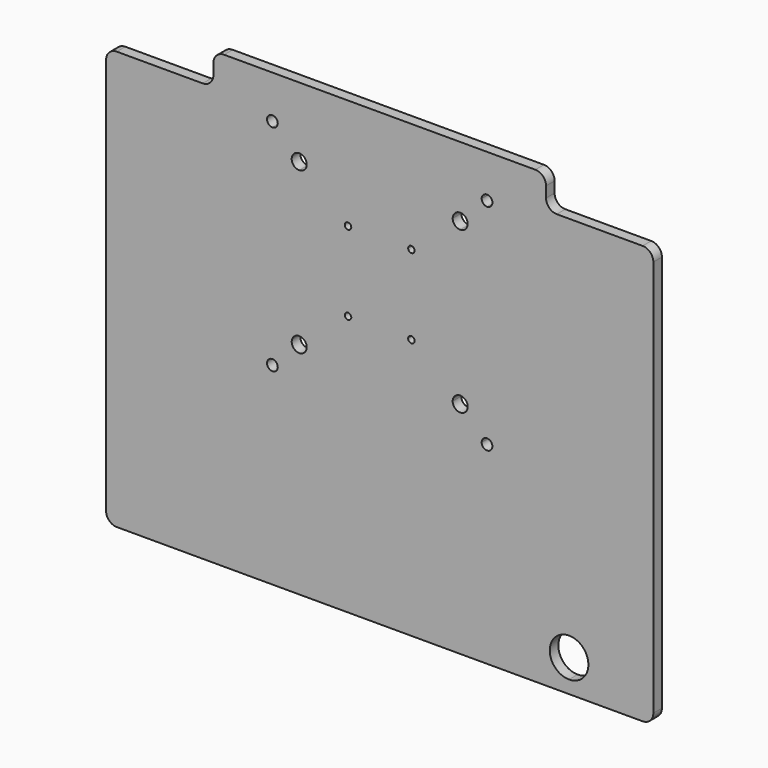
from build123d import *

# Parameters (mm, degrees)
F1_DEPTH = 5


with BuildPart() as f1:
    # F0 (on Front) → F1 (new body)
    with BuildSketch(Plane.XZ):
        with BuildLine():
            Line((88.225863874, -105), (122.5, -105))
            ThreePointArc((122.5, -105), (126.0355339059, -103.5355339059), (127.5, -100))
            Line((127.5, -100), (127.5, 85))
            ThreePointArc((127.5, 85), (126.0355339059, 88.5355339059), (122.5, 90))
            Line((122.5, 90), (82.5, 90))
            ThreePointArc((82.5, 90), (78.9644660941, 91.4644660941), (77.5, 95))
            Line((77.5, 95), (77.5, 100))
            ThreePointArc((77.5, 100), (76.0355339059, 103.5355339059), (72.5, 105))
            Line((72.5, 105), (0, 105))
            Line((0, 105), (-72.5, 105))
            ThreePointArc((-72.5, 105), (-76.0355339059, 103.5355339059), (-77.5, 100))
            Line((-77.5, 100), (-77.5, 95))
            ThreePointArc((-77.5, 95), (-78.9644660941, 91.4644660941), (-82.5, 90))
            Line((-82.5, 90), (-122.5, 90))
            ThreePointArc((-122.5, 90), (-126.0355339059, 88.5355339059), (-127.5, 85))
            Line((-127.5, 85), (-127.5, -100))
            ThreePointArc((-127.5, -100), (-126.0355339059, -103.5355339059), (-122.5, -105))
            Line((-122.5, -105), (88.225863874, -105))
        make_face()
        with BuildLine():
            ThreePointArc((97.225863874, -90), (94.5898249046, -96.3639610307), (88.225863874, -99))
            ThreePointArc((88.225863874, -99), (81.8619028433, -83.6360389693), (97.225863874, -90))
        make_face(mode=Mode.SUBTRACT)
        with BuildLine():
            Line((-47.5, 85), (0, 85))
            Line((0, 85), (47.5, 85))
            ThreePointArc((47.5, 85), (50, 87.5), (52.5, 85))
            ThreePointArc((52.5, 85), (51.767766953, 83.232233047), (50, 82.5))
            Line((50, 82.5), (50, -12.5))
            ThreePointArc((50, -12.5), (51.767766953, -13.232233047), (52.5, -15))
            ThreePointArc((52.5, -15), (50, -17.5), (47.5, -15))
            Line((47.5, -15), (-47.5, -15))
            ThreePointArc((-47.5, -15), (-51.767766953, -16.767766953), (-50, -12.5))
            Line((-50, -12.5), (-50, 82.5))
            ThreePointArc((-50, 82.5), (-51.767766953, 86.767766953), (-47.5, 85))
        make_face(mode=Mode.SUBTRACT)
        with BuildLine():
            Line((47.5, 85), (0, 85))
            Line((0, 85), (-47.5, 85))
            ThreePointArc((-47.5, 85), (-48.232233047, 83.232233047), (-50, 82.5))
            Line((-50, 82.5), (-50, -12.5))
            ThreePointArc((-50, -12.5), (-48.232233047, -13.232233047), (-47.5, -15))
            Line((-47.5, -15), (47.5, -15))
            ThreePointArc((47.5, -15), (48.232233047, -13.232233047), (50, -12.5))
            Line((50, -12.5), (50, 82.5))
            ThreePointArc((50, 82.5), (48.232233047, 83.232233047), (47.5, 85))
        make_face()
        with BuildLine():
            Line((34, -2.5), (-34, -2.5))
            ThreePointArc((-34, -2.5), (-39.9748737342, -4.9748737342), (-37.5, 1))
            Line((-37.5, 1), (-37.5, 69))
            ThreePointArc((-37.5, 69), (-39.9748737342, 74.9748737342), (-34, 72.5))
            Line((-34, 72.5), (34, 72.5))
            ThreePointArc((34, 72.5), (37.5, 76), (41, 72.5))
            ThreePointArc((41, 72.5), (39.9748737342, 70.0251262658), (37.5, 69))
            Line((37.5, 69), (37.5, 1))
            ThreePointArc((37.5, 1), (39.9748737342, -0.0251262658), (41, -2.5))
            ThreePointArc((41, -2.5), (37.5, -6), (34, -2.5))
        make_face(mode=Mode.SUBTRACT)
        with BuildLine():
            ThreePointArc((-37.5, 1), (-35.0251262658, -0.0251262658), (-34, -2.5))
            Line((-34, -2.5), (34, -2.5))
            ThreePointArc((34, -2.5), (35.0251262658, -0.0251262658), (37.5, 1))
            Line((37.5, 1), (37.5, 69))
            ThreePointArc((37.5, 69), (35.0251262658, 70.0251262658), (34, 72.5))
            Line((34, 72.5), (-34, 72.5))
            ThreePointArc((-34, 72.5), (-35.0251262658, 70.0251262658), (-37.5, 69))
            Line((-37.5, 69), (-37.5, 1))
        make_face()
        with BuildLine():
            Line((13.25, 16.5), (-13.25, 16.5))
            ThreePointArc((-13.25, 16.5), (-15.8106601718, 15.4393398282), (-14.75, 18))
            Line((-14.75, 18), (-14.75, 52))
            ThreePointArc((-14.75, 52), (-15.8106601718, 54.5606601718), (-13.25, 53.5))
            Line((-13.25, 53.5), (13.25, 53.5))
            ThreePointArc((13.25, 53.5), (14.75, 55), (16.25, 53.5))
            ThreePointArc((16.25, 53.5), (15.8106601718, 52.4393398282), (14.75, 52))
            Line((14.75, 52), (14.75, 18))
            ThreePointArc((14.75, 18), (15.8106601718, 17.5606601718), (16.25, 16.5))
            ThreePointArc((16.25, 16.5), (14.75, 15), (13.25, 16.5))
        make_face(mode=Mode.SUBTRACT)
        with BuildLine():
            ThreePointArc((-14.75, 18), (-13.6893398282, 17.5606601718), (-13.25, 16.5))
            Line((-13.25, 16.5), (13.25, 16.5))
            ThreePointArc((13.25, 16.5), (13.6893398282, 17.5606601718), (14.75, 18))
            Line((14.75, 18), (14.75, 52))
            ThreePointArc((14.75, 52), (13.6893398282, 52.4393398282), (13.25, 53.5))
            Line((13.25, 53.5), (-13.25, 53.5))
            ThreePointArc((-13.25, 53.5), (-13.6893398282, 52.4393398282), (-14.75, 52))
            Line((-14.75, 52), (-14.75, 18))
        make_face()
    extrude(amount=F1_DEPTH)


solid = f1.part
